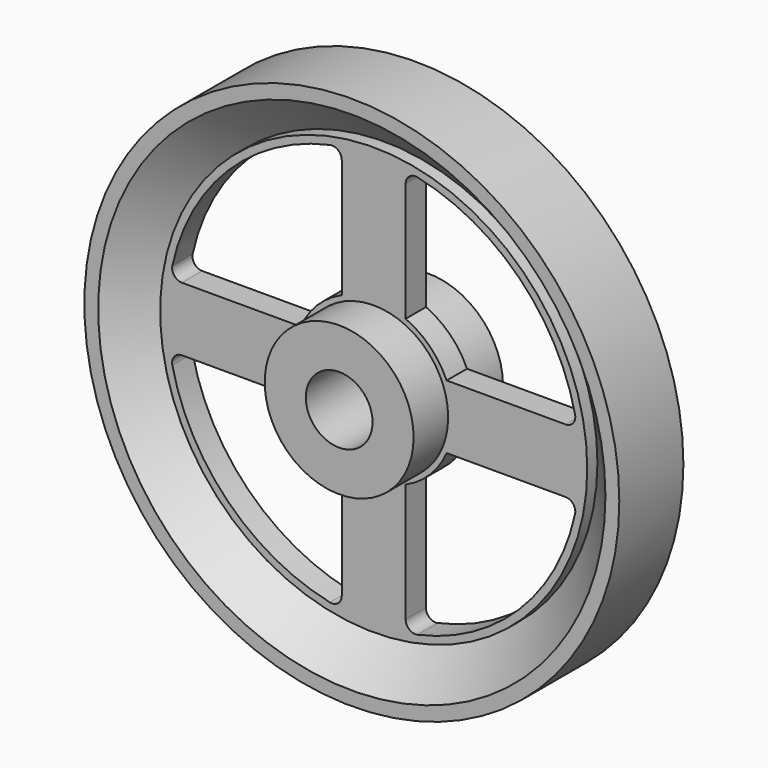
from build123d import *

# Parameters (mm, degrees)
F0_R     = 109.2819211761
F0_R_2   = 38.0943795336
F1_DEPTH = 6.5
F0_R_3   = 17.0786254613
F2_DEPTH = 28.6
F3_R     = 130.7
F3_R_2   = 109.285
F4_DEPTH = 20.5
F5_SIZE  = 20.49999
F3_R_3   = 136.88
F6_DEPTH = 20.5


# Not quite as in the source:
# - a fillet or chamfer is up to 0.001 mm smaller than in the source, because OpenCascade refuses the exact size


with BuildPart() as f1:
    # F0 (on Front) → F1 (new body, symmetric)
    with BuildSketch(Plane.XZ):
        Circle(F0_R)
        with BuildLine():
            Line((-98.1561071561, -16.35), (-37.3311538661, -16.35))
            ThreePointArc((-37.3311538661, -16.35), (-28.8178551334, -28.8178551334), (-16.35, -37.3311538661))
            Line((-16.35, -37.3311538661), (-16.35, -98.1561071561))
            ThreePointArc((-16.35, -98.1561071561), (-18.2126065992, -102.0492758718), (-22.4127050594, -103.0418678908))
            ThreePointArc((-22.4127050594, -103.0418678908), (-74.5652596271, -74.5652596271), (-103.0418678908, -22.4127050594))
            ThreePointArc((-103.0418678908, -22.4127050594), (-102.0492758718, -18.2126065992), (-98.1561071561, -16.35))
        make_face(mode=Mode.SUBTRACT)
        Circle(F0_R_2, mode=Mode.SUBTRACT)
        with BuildLine():
            ThreePointArc((103.0418678908, -22.4127050594), (74.5652596271, -74.5652596271), (22.4127050594, -103.0418678908))
            ThreePointArc((22.4127050594, -103.0418678908), (18.2126065992, -102.0492758718), (16.35, -98.1561071561))
            Line((16.35, -98.1561071561), (16.35, -37.3311538661))
            ThreePointArc((16.35, -37.3311538661), (28.8178551334, -28.8178551334), (37.3311538661, -16.35))
            Line((37.3311538661, -16.35), (98.1561071561, -16.35))
            ThreePointArc((98.1561071561, -16.35), (102.0492758718, -18.2126065992), (103.0418678908, -22.4127050594))
        make_face(mode=Mode.SUBTRACT)
        with BuildLine():
            Line((-16.35, 98.1561071561), (-16.35, 37.3311538661))
            ThreePointArc((-16.35, 37.3311538661), (-28.8178551334, 28.8178551334), (-37.3311538661, 16.35))
            Line((-37.3311538661, 16.35), (-98.1561071561, 16.35))
            ThreePointArc((-98.1561071561, 16.35), (-102.0492758718, 18.2126065992), (-103.0418678908, 22.4127050594))
            ThreePointArc((-103.0418678908, 22.4127050594), (-74.5652596271, 74.5652596271), (-22.4127050594, 103.0418678908))
            ThreePointArc((-22.4127050594, 103.0418678908), (-18.2126065992, 102.0492758718), (-16.35, 98.1561071561))
        make_face(mode=Mode.SUBTRACT)
        with BuildLine():
            Line((98.1561071561, 16.35), (37.3311538661, 16.35))
            ThreePointArc((37.3311538661, 16.35), (28.8178551334, 28.8178551334), (16.35, 37.3311538661))
            Line((16.35, 37.3311538661), (16.35, 98.1561071561))
            ThreePointArc((16.35, 98.1561071561), (18.2126065992, 102.0492758718), (22.4127050594, 103.0418678908))
            ThreePointArc((22.4127050594, 103.0418678908), (74.5652596271, 74.5652596271), (103.0418678908, 22.4127050594))
            ThreePointArc((103.0418678908, 22.4127050594), (102.0492758718, 18.2126065992), (98.1561071561, 16.35))
        make_face(mode=Mode.SUBTRACT)
    extrude(amount=F1_DEPTH, both=True)

    # F0 (on Front) → F2 (join, symmetric)
    with BuildSketch(Plane.XZ):
        Circle(F0_R_2)
        Circle(F0_R_3, mode=Mode.SUBTRACT)
    extrude(amount=F2_DEPTH, both=True)


with BuildPart() as f4:
    # F3 (on face) → F4 (new body, symmetric)
    with BuildSketch(Plane.XZ):
        Circle(F3_R)
        Circle(F3_R_2, mode=Mode.SUBTRACT)
    extrude(amount=F4_DEPTH, both=True)

    # F5 (size 20.5 in the source; OpenCascade refuses exactly that, so slightly less here)
    f5_edges = [f4.edges().sort_by_distance(p)[0] for p in [
        (-109.285, -20.5, 0),
        (109.285, 0, 0),
        (-109.285, 20.5, 0),
    ]]
    chamfer(f5_edges, length=F5_SIZE)

    # F3 (on face) → F6 (join, symmetric)
    with BuildSketch(Plane.XZ):
        Circle(F3_R_3)
        Circle(F3_R, mode=Mode.SUBTRACT)
    extrude(amount=F6_DEPTH, both=True)


solid = Compound([f1.part, f4.part])
